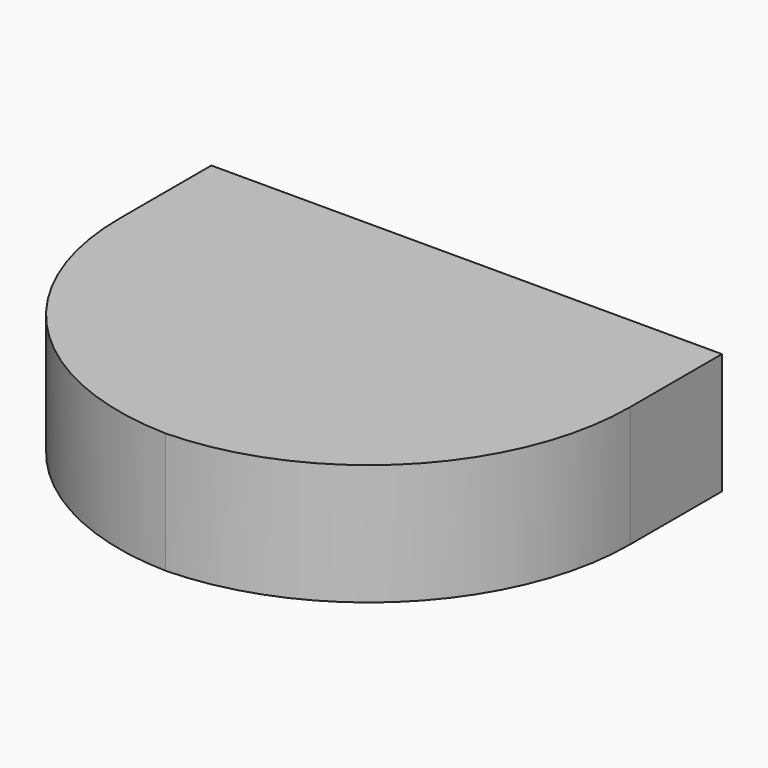
from build123d import *

# Parameters (mm, degrees)
F0_W        = 76
F0_H        = 56
F1_DEPTH    = 18
F2_T1_DEPTH = 212.344191771


# Not quite as in the source:
# - a fillet or chamfer that OpenCascade refuses, or shapes differently, is made with other operations: its cross-section is extruded or revolved along the edge and cut away or added


with BuildPart() as f1:
    # F0 (on Top) → F1 (new body)
    with BuildSketch(Plane.XY):
        with Locations((2.4067710042, -5.2896709442)):
            Rectangle(F0_W, F0_H)
    extrude(amount=F1_DEPTH)

    # F2: fillet of radius 38.8688383542 on 2 edges, made by hand

    # F2_s2 → F2_t1 (cut)
    with BuildSketch(Plane.XY.offset(-97.1720958855)):
        with BuildLine():
            ThreePointArc((-35.5932289958, 5.57916741), (-24.2088098187, -21.9052517671), (3.2756093584, -33.2896709442))
            Line((3.2756093584, -33.2896709442), (-35.5932289958, -33.2896709442))
            Line((-35.5932289958, -33.2896709442), (-35.5932289958, 5.57916741))
        make_face()
        with BuildLine():
            ThreePointArc((40.4067710042, 5.57916741), (29.0223518271, -21.9052517671), (1.53793265, -33.2896709442))
            Line((1.53793265, -33.2896709442), (40.4067710042, -33.2896709442))
            Line((40.4067710042, -33.2896709442), (40.4067710042, 5.57916741))
        make_face()
    extrude(amount=F2_T1_DEPTH, mode=Mode.SUBTRACT)


solid = f1.part
